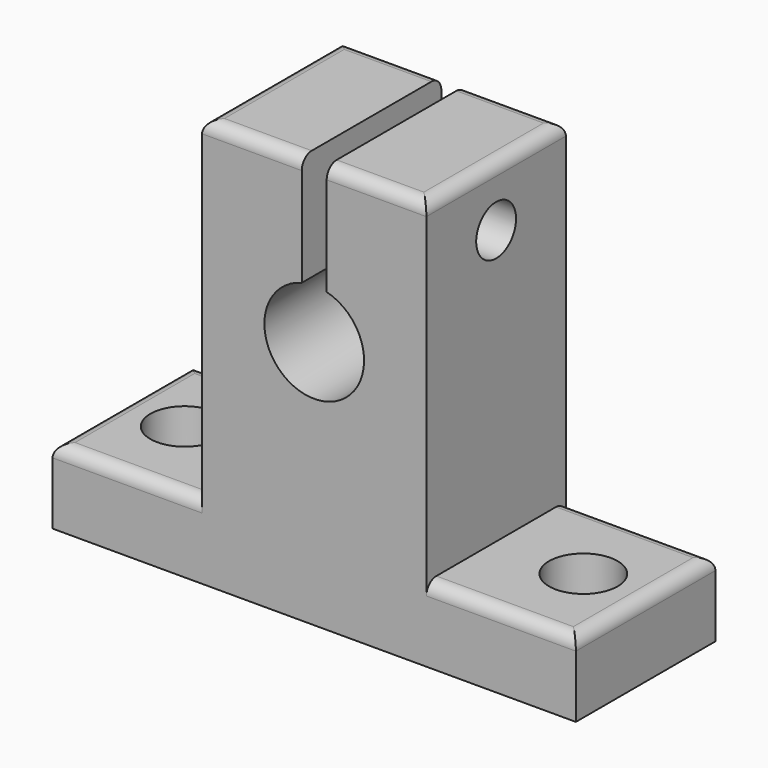
from build123d import *

# Parameters (mm, degrees)
F1_DEPTH      = 14
F2_R          = 2.75
F3_DEPTH      = 6
F4_R          = 1
F5_R          = 2
F6_DEPTH      = 10
F6_DEPTH_BACK = 9
F7_R          = 0.5


with BuildPart() as f1:
    # F0 (on Front) → F1 (new body)
    with BuildSketch(Plane.XZ):
        with BuildLine():
            Line((-9, 6), (-21, 6))
            Line((-21, 6), (-21, 0))
            Line((-21, 0), (21, 0))
            Line((21, 0), (21, 6))
            Line((21, 6), (9, 6))
            Line((9, 6), (9, 32.8))
            Line((9, 32.8), (1, 32.8))
            Line((1, 32.8), (1, 23.8729833462))
            ThreePointArc((1, 23.8729833462), (0, 16), (-1, 23.8729833462))
            Line((-1, 23.8729833462), (-1, 32.8))
            Line((-1, 32.8), (-9, 32.8))
            Line((-9, 32.8), (-9, 6))
        make_face()
    extrude(amount=F1_DEPTH)

    # F2 (on Top) → F3 (cut)
    with BuildSketch(Plane.XY):
        with Locations((16, -7)):
            Circle(F2_R)
        with Locations((-16, -7)):
            Circle(F2_R)
    extrude(amount=F3_DEPTH, mode=Mode.SUBTRACT)

    # F4
    f4_edges = [f1.edges().sort_by_distance(p)[0] for p in [
        (-21, -7, 6),
        (-15, 0, 6),
        (-15, -14, 6),
        (15, -14, 6),
        (21, -7, 6),
        (15, 0, 6),
        (-9, -7, 32.8),
        (9, -7, 32.8),
        (5, 0, 32.8),
        (-5, 0, 32.8),
        (-5, -14, 32.8),
        (5, -14, 32.8),
    ]]
    fillet(f4_edges, radius=F4_R)

    # F5 (on Right) → F6 (cut, two sides)
    with BuildSketch(Plane.YZ) as f6_sk:
        with Locations((-7, 28)):
            Circle(F5_R)
    extrude(amount=-F6_DEPTH, mode=Mode.SUBTRACT)
    extrude(f6_sk.sketch, amount=F6_DEPTH_BACK, mode=Mode.SUBTRACT)

    # F7
    f7_edges = [f1.edges().sort_by_distance(p)[0] for p in [
        (1, -9, 28),
        (-9, -9, 28),
        (-1, -9, 28),
    ]]
    fillet(f7_edges, radius=F7_R)


solid = f1.part
